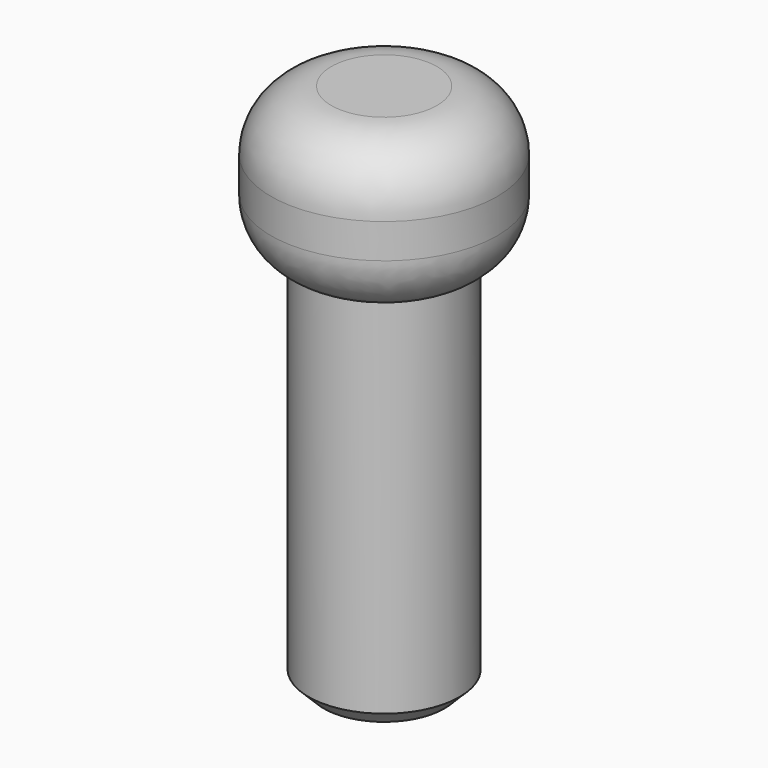
from build123d import *

# Parameters (mm, degrees)
F3_SIZE  = 1.27
F5_D     = 5.1054
F5_DEPTH = 29.21
F5_TIP   = 1.5338169022


# Not quite as in the source:
# - a fillet or chamfer that OpenCascade refuses, or shapes differently, is made with other operations: its cross-section is extruded or revolved along the edge and cut away or added


with BuildPart() as f1:
    # F0 (on Front) → F1 (revolve)
    with BuildSketch(Plane.XZ):
        Polygon((9.525, 12.7), (0, 12.7), (0, -31.75), (6.35, -31.75), (6.35, 0), (9.525, 0), align=None)
    revolve(axis=Axis((0, 0, -3.4719856316), (0, 0, -1)))

    # F2: fillet of radius 5.08 on 2 edges, made by hand

    # F2_s1 → F2_t2 (revolve, cut)
    with BuildSketch(Plane.XZ):
        with BuildLine():
            ThreePointArc((4.445, 12.7), (8.0371024484, 11.2121024484), (9.525, 7.62))
            Line((9.525, 7.62), (9.525, 12.7))
            Line((9.525, 12.7), (4.445, 12.7))
        make_face()
    revolve(axis=Axis((0, 0, 12.7), (0, 0, -1)), mode=Mode.SUBTRACT)

    # F2_s3 → F2_t4 (revolve, cut)
    with BuildSketch(Plane.XZ):
        with BuildLine():
            ThreePointArc((6.35, 0), (8.6571134838, 1.8694797079), (9.525, 4.7092860393))
            Line((9.525, 4.7092860393), (9.525, 0))
            Line((9.525, 0), (6.35, 0))
        make_face()
    revolve(axis=Axis((0, 0, 0), (0, 0, -1)), mode=Mode.SUBTRACT)

    # F3
    f3_edges = [f1.edges().sort_by_distance(p)[0] for p in [
        (-6.35, 0, -31.75),
    ]]
    chamfer(f3_edges, length=F3_SIZE)

    # F5
    with Locations(Plane(origin=(0, 0, -31.75), x_dir=(1, 0, 0), z_dir=(0, 0, -1))):
        with Locations((0, 0)):
            Hole(F5_D / 2, depth=F5_DEPTH)
            with Locations((0, 0, -(F5_DEPTH + F5_TIP / 2))):  # 118° drill point
                Cone(0, F5_D / 2, F5_TIP, mode=Mode.SUBTRACT)


solid = f1.part
